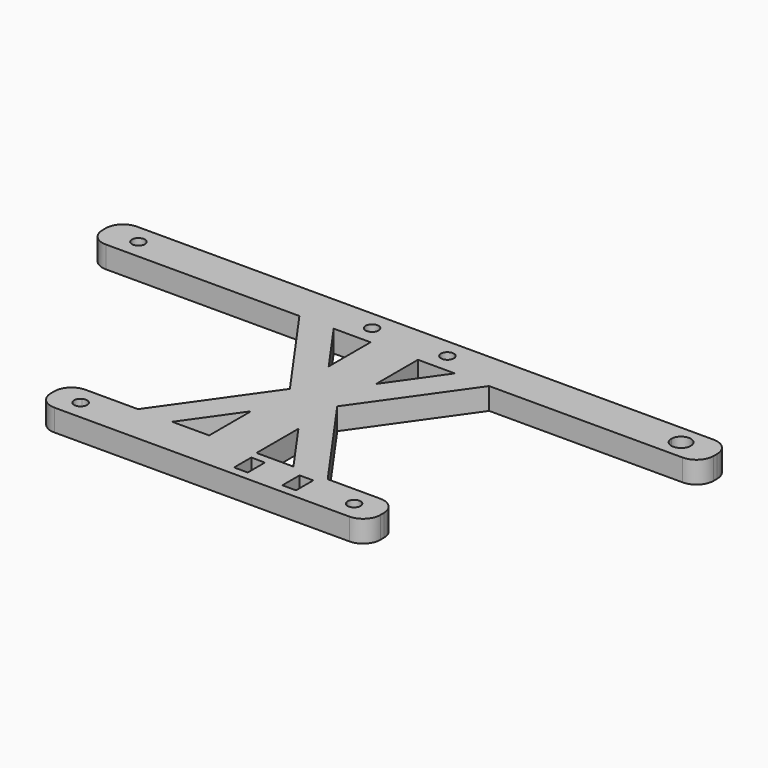
from build123d import *

# Parameters (mm, degrees)
F1_DEPTH = 5.08
F2_R     = 4


# Not quite as in the source:
# - a feature names something its author has since deleted; it is built from what else it names


with BuildPart() as f1:
    # F0 (on Top) → F1 (new body)
    with BuildSketch(Plane.XY):
        with BuildLine():
            Line((0.6656670719, 55.8519247654), (-50.5843329281, 55.8519247654))
            ThreePointArc((-50.5843329281, 55.8519247654), (-50.7903791398, 55.0931866065), (-51.3519110531, 54.5428952787))
            Line((-51.3519110531, 54.5428952787), (-49.566514597, 51.3519247654))
            Line((-49.566514597, 51.3519247654), (-11.1088099211, 51.3519247654))
            Line((-11.1088099211, 51.3519247654), (-3.1543997556, 51.3519247654))
            Line((-3.1543997556, 51.3519247654), (5.4156670719, 51.3519247654))
            Line((5.4156670719, 51.3519247654), (10.9156670719, 51.3519247654))
            Line((10.9156670719, 51.3519247654), (10.9156670719, 55.8519247654))
            Line((10.9156670719, 55.8519247654), (3.6656670719, 55.8519247654))
            ThreePointArc((3.6656670719, 55.8519247654), (2.1656670719, 54.3519247654), (0.6656670719, 55.8519247654))
        make_face()
        with BuildLine():
            Line((-11.1088099211, 4.5), (-23.3521512592, 4.5))
            Line((-23.3521512592, 4.5), (-21.5667548031, 1.3090294867))
            ThreePointArc((-21.5667548031, 1.3090294867), (-20.0755947692, 1.2939537883), (-19.3343329281, 0))
            Line((-19.3343329281, 0), (10.9156670719, 0))
            Line((10.9156670719, 0), (10.9156670719, 4.5))
            Line((10.9156670719, 4.5), (5.4156670719, 4.5))
            Line((5.4156670719, 4.5), (-3.1543997556, 4.5))
            Line((-3.1543997556, 4.5), (-11.1088099211, 4.5))
        make_face()
        with BuildLine():
            ThreePointArc((-51.3519110531, 54.5428952787), (-53.3782867164, 56.6106629243), (-50.5843329281, 55.8519247654))
            Line((-50.5843329281, 55.8519247654), (0.6656670719, 55.8519247654))
            ThreePointArc((0.6656670719, 55.8519247654), (2.1656670719, 57.3519247654), (3.6656670719, 55.8519247654))
            Line((3.6656670719, 55.8519247654), (10.9156670719, 55.8519247654))
            Line((10.9156670719, 55.8519247654), (18.1656670719, 55.8519247654))
            ThreePointArc((18.1656670719, 55.8519247654), (19.6656670719, 57.3519247654), (21.1656670719, 55.8519247654))
            Line((21.1656670719, 55.8519247654), (71.6656670719, 55.8519247654))
            ThreePointArc((71.6656670719, 55.8519247654), (73.9156670719, 58.1019247654), (76.1656670719, 55.8519247654))
            ThreePointArc((76.1656670719, 55.8519247654), (75.0537743102, 53.910994083), (72.8170342594, 53.8883805354))
            Line((72.8170342594, 53.8883805354), (71.3978487408, 51.3519247654))
            Line((71.3978487408, 51.3519247654), (81.8841302488, 51.3519247654))
            Line((81.8841302488, 51.3519247654), (81.8841302488, 60.3519247654))
            Line((81.8841302488, 60.3519247654), (-60.052796105, 60.3519247654))
            Line((-60.052796105, 60.3519247654), (-60.052796105, 51.3519247654))
            Line((-60.052796105, 51.3519247654), (-49.566514597, 51.3519247654))
            Line((-49.566514597, 51.3519247654), (-51.3519110531, 54.5428952787))
        make_face()
        with BuildLine():
            Line((-21.5667548031, 1.3090294867), (-23.3521512592, 4.5))
            Line((-23.3521512592, 4.5), (-27.3365851734, 4.5))
            Line((-27.3365851734, 4.5), (-27.3365851734, -4.5))
            Line((-27.3365851734, -4.5), (49.1679193172, -4.5))
            Line((49.1679193172, -4.5), (49.1679193172, 4.5))
            Line((49.1679193172, 4.5), (45.183485403, 4.5))
            Line((45.183485403, 4.5), (43.3980889469, 1.3090294867))
            ThreePointArc((43.3980889469, 1.3090294867), (43.9596208602, 0.7587381589), (44.1656670719, 0))
            ThreePointArc((44.1656670719, 0), (42.6656670719, -1.5), (41.1656670719, 0))
            Line((41.1656670719, 0), (31.1806510627, 0))
            Line((31.1806510627, 0), (31.1806510627, -2.5))
            Line((31.1806510627, -2.5), (28.0056510627, -2.5))
            Line((28.0056510627, -2.5), (28.0056510627, 0))
            Line((28.0056510627, 0), (19.9686510627, 0))
            Line((19.9686510627, 0), (19.9686510627, -2.5))
            Line((19.9686510627, -2.5), (16.7936510627, -2.5))
            Line((16.7936510627, -2.5), (16.7936510627, 0))
            Line((16.7936510627, 0), (10.9156670719, 0))
            Line((10.9156670719, 0), (-19.3343329281, 0))
            ThreePointArc((-19.3343329281, 0), (-21.593071087, -1.2939537883), (-21.5667548031, 1.3090294867))
        make_face()
        with BuildLine():
            Line((10.9156670719, 4.5), (10.9156670719, 0))
            Line((10.9156670719, 0), (16.7936510627, 0))
            Line((16.7936510627, 0), (16.7936510627, 2.5))
            Line((16.7936510627, 2.5), (19.9686510627, 2.5))
            Line((19.9686510627, 2.5), (19.9686510627, 0))
            Line((19.9686510627, 0), (28.0056510627, 0))
            Line((28.0056510627, 0), (28.0056510627, 2.5))
            Line((28.0056510627, 2.5), (31.1806510627, 2.5))
            Line((31.1806510627, 2.5), (31.1806510627, 0))
            Line((31.1806510627, 0), (41.1656670719, 0))
            ThreePointArc((41.1656670719, 0), (41.906928913, 1.2939537883), (43.3980889469, 1.3090294867))
            Line((43.3980889469, 1.3090294867), (45.183485403, 4.5))
            Line((45.183485403, 4.5), (32.9401440649, 4.5))
            Line((32.9401440649, 4.5), (24.9857338994, 4.5))
            Line((24.9857338994, 4.5), (16.4156670719, 4.5))
            Line((16.4156670719, 4.5), (10.9156670719, 4.5))
        make_face()
        with BuildLine():
            Line((18.1656670719, 55.8519247654), (10.9156670719, 55.8519247654))
            Line((10.9156670719, 55.8519247654), (10.9156670719, 51.3519247654))
            Line((10.9156670719, 51.3519247654), (16.4156670719, 51.3519247654))
            Line((16.4156670719, 51.3519247654), (24.9857338994, 51.3519247654))
            Line((24.9857338994, 51.3519247654), (32.9401440649, 51.3519247654))
            Line((32.9401440649, 51.3519247654), (71.3978487408, 51.3519247654))
            Line((71.3978487408, 51.3519247654), (72.8170342594, 53.8883805354))
            ThreePointArc((72.8170342594, 53.8883805354), (71.9747363894, 54.7138175271), (71.6656670719, 55.8519247654))
            Line((71.6656670719, 55.8519247654), (21.1656670719, 55.8519247654))
            ThreePointArc((21.1656670719, 55.8519247654), (19.6656670719, 54.3519247654), (18.1656670719, 55.8519247654))
        make_face()
        Polygon((5.4156670719, 39.2025500407), (5.4156670719, 27.9259623827), (10.9156670719, 27.9259623827), (10.9156670719, 51.3519247654), (5.4156670719, 51.3519247654), align=None)
        Polygon((10.9156670719, 27.9259623827), (5.4156670719, 27.9259623827), (5.4156670719, 16.6493747247), (5.4156670719, 4.5), (10.9156670719, 4.5), align=None)
        Polygon((16.4156670719, 51.3519247654), (10.9156670719, 51.3519247654), (10.9156670719, 27.9259623827), (16.4156670719, 27.9259623827), (16.4156670719, 39.2025500407), align=None)
        Polygon((16.4156670719, 27.9259623827), (10.9156670719, 27.9259623827), (10.9156670719, 4.5), (16.4156670719, 4.5), (16.4156670719, 16.6493747247), align=None)
        Polygon((-3.1543997556, 51.3519247654), (-11.1088099211, 51.3519247654), (5.4156670719, 27.9259623827), (5.4156670719, 39.2025500407), align=None)
        Polygon((5.4156670719, 27.9259623827), (-11.1088099211, 4.5), (-3.1543997556, 4.5), (5.4156670719, 16.6493747247), align=None)
        Polygon((32.9401440649, 4.5), (16.4156670719, 27.9259623827), (16.4156670719, 16.6493747247), (24.9857338994, 4.5), align=None)
        Polygon((16.4156670719, 39.2025500407), (16.4156670719, 27.9259623827), (32.9401440649, 51.3519247654), (24.9857338994, 51.3519247654), align=None)
    extrude(amount=F1_DEPTH)

    # F2
    f2_edges = [f1.edges().sort_by_distance(p)[0] for p in [
        (-60.052796, 60.351925, 2.54),
        (-60.052796, 51.351925, 2.54),
        (81.88413, 60.351925, 2.54),
        (81.88413, 51.351925, 2.54),
        (49.167919, 4.5, 2.54),
        (49.167919, -4.5, 2.54),
        (-27.336585, 4.5, 2.54),
        (-27.336585, -4.5, 2.54),
    ]]
    fillet(f2_edges, radius=F2_R)


solid = f1.part
